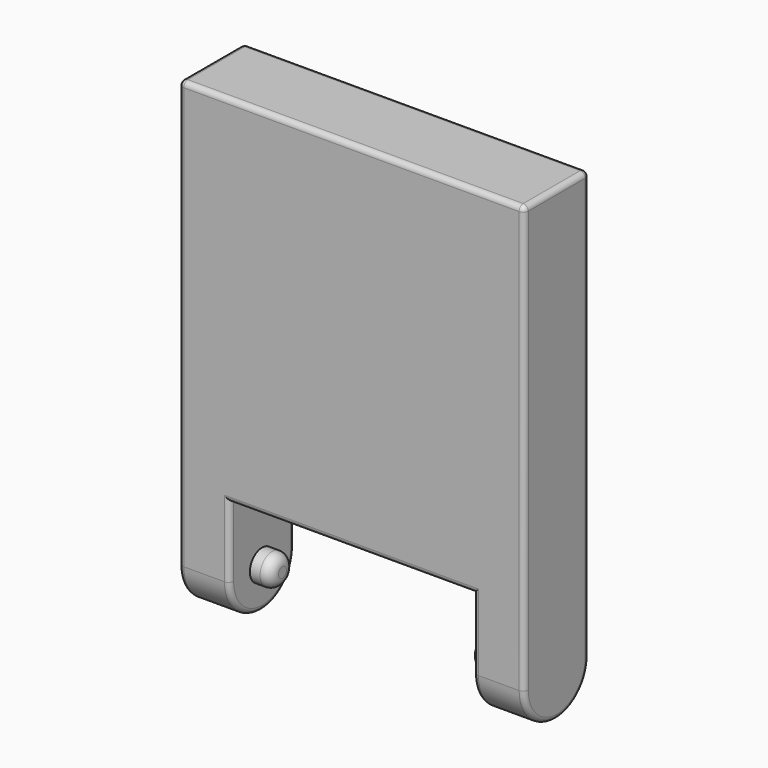
from build123d import *

# Parameters (mm, degrees)
F0_W     = 34
F0_H     = 35
F1_DEPTH = 8
F2_W     = 5
F2_H     = 8
F3_DEPTH = 11
F4_R     = 3.99999
F6_DEPTH = 2
F7_R     = 1
F9_DEPTH = 2
F10_R    = 1
F11_R    = 0.5


# Not quite as in the source:
# - a fillet or chamfer is up to 0.001 mm smaller than in the source, because OpenCascade refuses the exact size


with BuildPart() as f1:
    # F0 (on Front) → F1 (new body)
    with BuildSketch(Plane.XZ):
        with Locations((17, 17.5)):
            Rectangle(F0_W, F0_H)
    extrude(amount=-F1_DEPTH)

    # F2 (on face) → F3 (join)
    with BuildSketch(Plane(origin=(0, 0, 0), x_dir=(1, 0, 0), z_dir=(0, 0, -1))):
        with Locations((31.5, -4)):
            Rectangle(F2_W, F2_H)
        with Locations((2.5, -4)):
            Rectangle(F2_W, F2_H)
    extrude(amount=F3_DEPTH)

    # F4 (radius 4 in the source; OpenCascade refuses exactly that, so slightly less here)
    f4_edges = [f1.edges().sort_by_distance(p)[0] for p in [
        (2.5, 0, -11),
        (2.5, 8, -11),
        (31.5, 8, -11),
        (31.5, 0, -11),
    ]]
    fillet(f4_edges, radius=F4_R)

    # F5 (on face) → F6 (join)
    with BuildSketch(Plane(origin=(29, 0, 0), x_dir=(0, -1, 0), z_dir=(-1, 0, 0))):
        with BuildLine():
            Line((-5.027864045, -7), (-2.027864045, -7))
            ThreePointArc((-2.027864045, -7), (-3.527864045, -5.5), (-5.027864045, -7))
        make_face()
        with BuildLine():
            ThreePointArc((-5.027864045, -7), (-3.527864045, -8.5), (-2.027864045, -7))
            Line((-2.027864045, -7), (-5.027864045, -7))
        make_face()
    extrude(amount=F6_DEPTH)

    # F7
    f7_edges = [f1.edges().sort_by_distance(p)[0] for p in [
        (27, 2.027864, -7),
    ]]
    fillet(f7_edges, radius=F7_R)

    # F8 (on face) → F9 (join)
    with BuildSketch(Plane.YZ.offset(5)):
        with BuildLine():
            Line((2.5, -7), (5.5, -7))
            ThreePointArc((5.5, -7), (4, -5.5), (2.5, -7))
        make_face()
        with BuildLine():
            ThreePointArc((2.5, -7), (4, -8.5), (5.5, -7))
            Line((5.5, -7), (2.5, -7))
        make_face()
    extrude(amount=F9_DEPTH)

    # F10
    f10_edges = [f1.edges().sort_by_distance(p)[0] for p in [
        (7, 5.5, -7),
    ]]
    fillet(f10_edges, radius=F10_R)

    # F11
    f11_edges = [f1.edges().sort_by_distance(p)[0] for p in [
        (0, 0, 13.999995),
        (2.5, 0, -7.00001),
        (17, 0, 35),
        (5, 0, -3.500005),
        (34, 0, 13.999995),
        (17, 0, 0),
        (31.5, 0, -7.00001),
        (29, 0, -3.500005),
        (0, 8, 13.999995),
        (2.5, 8, -7.00001),
        (17, 8, 35),
        (5, 8, -3.500005),
        (34, 8, 13.999995),
        (17, 8, 0),
        (31.5, 8, -7.00001),
        (29, 8, -3.500005),
        (34, 4, 35),
        (0, 4, 35),
    ]]
    fillet(f11_edges, radius=F11_R)


solid = f1.part
